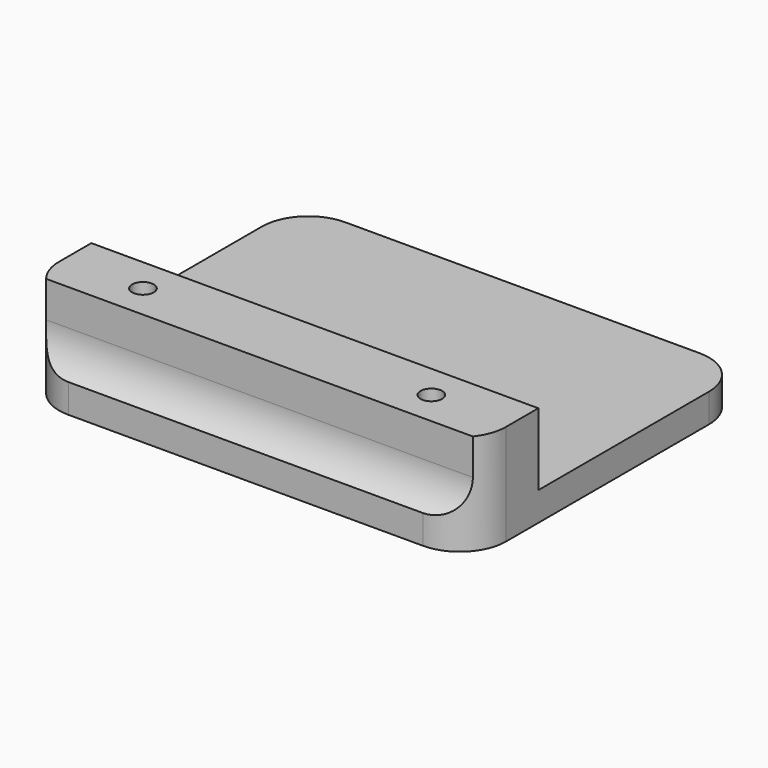
from build123d import *

# Parameters (mm, degrees)
F0_W        = 49.2125
F0_H        = 38.1
F1_DEPTH    = 3.175
F2_W        = 49.2125
F2_H        = 7.62
F3_DEPTH    = 7.9375
F4_R        = 1.190625
F5_DEPTH    = 25.4
F6_T1_DEPTH = 49.2125
F7_R        = 5.08


# Not quite as in the source:
# - a fillet or chamfer that OpenCascade refuses, or shapes differently, is made with other operations: its cross-section is extruded or revolved along the edge and cut away or added


with BuildPart() as f1:
    # F0 (on Top) → F1 (new body)
    with BuildSketch(Plane.XY):
        Rectangle(F0_W, F0_H)
    extrude(amount=F1_DEPTH)

    # F2 (on face) → F3 (join)
    with BuildSketch(Plane.XY.offset(3.175)):
        with Locations((0, -13.335)):
            Rectangle(F2_W, F2_H)
    extrude(amount=F3_DEPTH)

    # F4 (on face) → F5 (cut)
    with BuildSketch(Plane.XY.offset(11.1125)):
        with Locations((-15.875, -13.335)):
            Circle(F4_R)
        with Locations((15.875, -13.335)):
            Circle(F4_R)
    extrude(amount=-F5_DEPTH, mode=Mode.SUBTRACT)

    # F6: fillet of radius 5.08 on 1 edges, made by hand

    # F6_s2 → F6_t1 (join)
    with BuildSketch(Plane.YZ.offset(-24.60625)):
        with BuildLine():
            ThreePointArc((-19.05, 3.175), (-17.6459498802, 4.9408692034), (-17.145, 7.140573729))
            Line((-17.145, 7.140573729), (-17.145, 3.175))
            Line((-17.145, 3.175), (-19.05, 3.175))
        make_face()
    extrude(amount=F6_T1_DEPTH)

    # F7
    f7_edges = [f1.edges().sort_by_distance(p)[0] for p in [
        (-24.60625, -19.05, 1.5875),
        (24.60625, -19.05, 1.5875),
        (24.60625, 19.05, 1.5875),
        (-24.60625, 19.05, 1.5875),
    ]]
    fillet(f7_edges, radius=F7_R)


solid = f1.part
